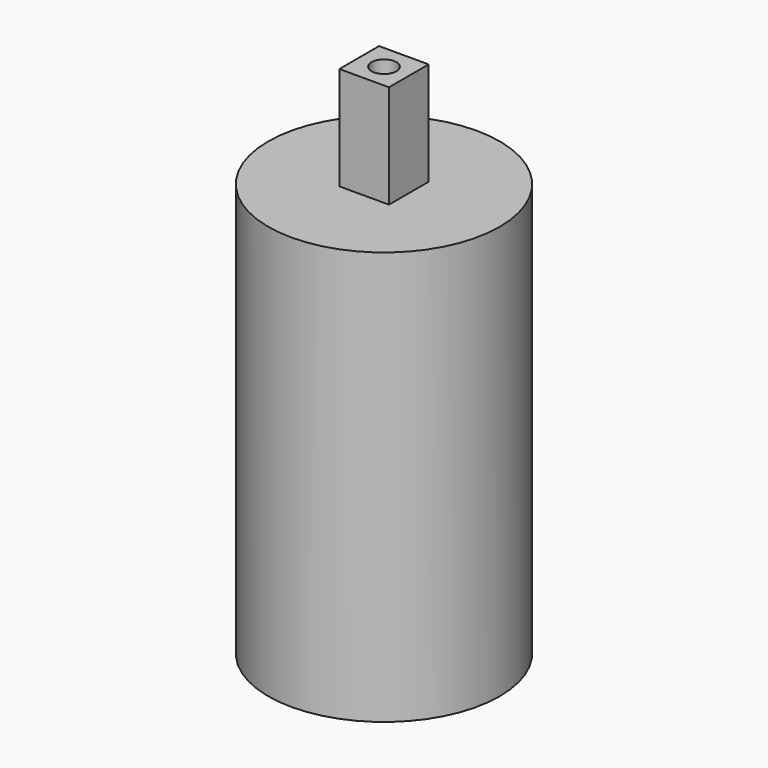
from build123d import *

# Parameters (mm, degrees)
F0_R     = 28
F0_R_2   = 25
F1_DEPTH = 100
F0_W     = 12
F0_H     = 12
F2_DEPTH = 10
F3_R     = 25
F3_W     = 12
F3_H     = 12
F4_DEPTH = 10
F0_R_3   = 3
F5_DEPTH = 10
F6_DEPTH = 125


with BuildPart() as f1:
    # F0 (on Top) → F1 (new body)
    with BuildSketch(Plane.XY):
        Circle(F0_R)
        Circle(F0_R_2, mode=Mode.SUBTRACT)
    extrude(amount=F1_DEPTH)

    # F0 (on Top) → F2 (join)
    with BuildSketch(Plane.XY):
        Circle(F0_R_2)
        Rectangle(F0_W, F0_H, mode=Mode.SUBTRACT)
    extrude(amount=F2_DEPTH)

    # F3 (on face) → F4 (join)
    with BuildSketch(Plane.XY.offset(100)):
        Circle(F3_R)
        Rectangle(F3_W, F3_H, mode=Mode.SUBTRACT)
    extrude(amount=-F4_DEPTH)


with BuildPart() as f5:
    # F0 (on Top) → F5 (new body)
    with BuildSketch(Plane.XY):
        Rectangle(F0_W, F0_H)
        Circle(F0_R_3, mode=Mode.SUBTRACT)
    extrude(amount=F5_DEPTH)

    # F0 (on Top) → F6 (join)
    with BuildSketch(Plane.XY):
        Rectangle(F0_W, F0_H)
        Circle(F0_R_3, mode=Mode.SUBTRACT)
    extrude(amount=F6_DEPTH)


solid = Compound([f1.part, f5.part])
